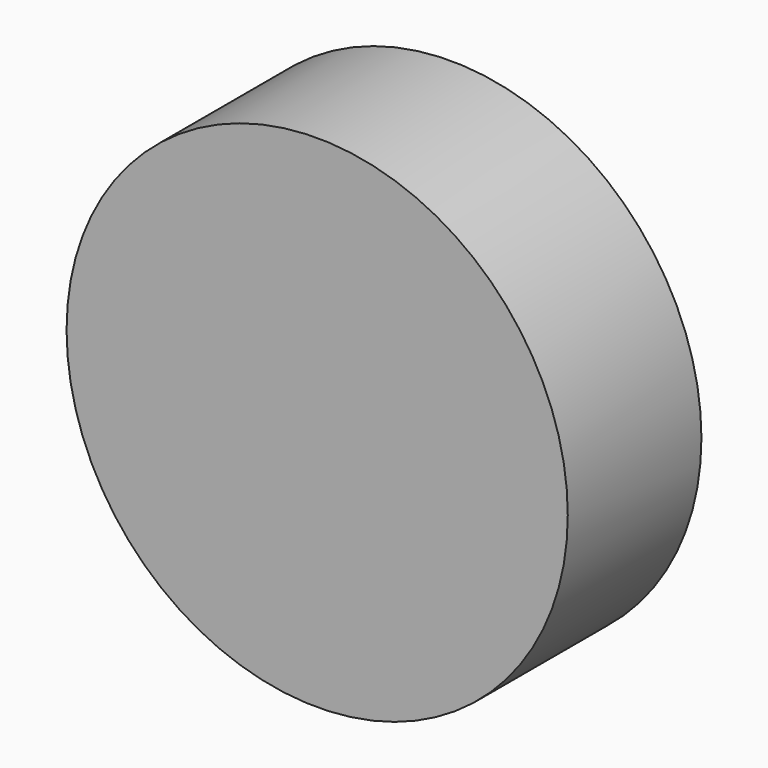
from build123d import *

# Parameters (mm, degrees)
F0_R     = 38.1
F1_DEPTH = 25.4


# Not quite as in the source:
# - the program builds the solid bodies; features that only make, move or delete a surface that nothing else refers to are left out


with BuildPart() as f1:
    # F0 (on Front) → F1 (new body)
    with BuildSketch(Plane.XZ):
        Circle(F0_R)
    extrude(amount=F1_DEPTH)


solid = f1.part
